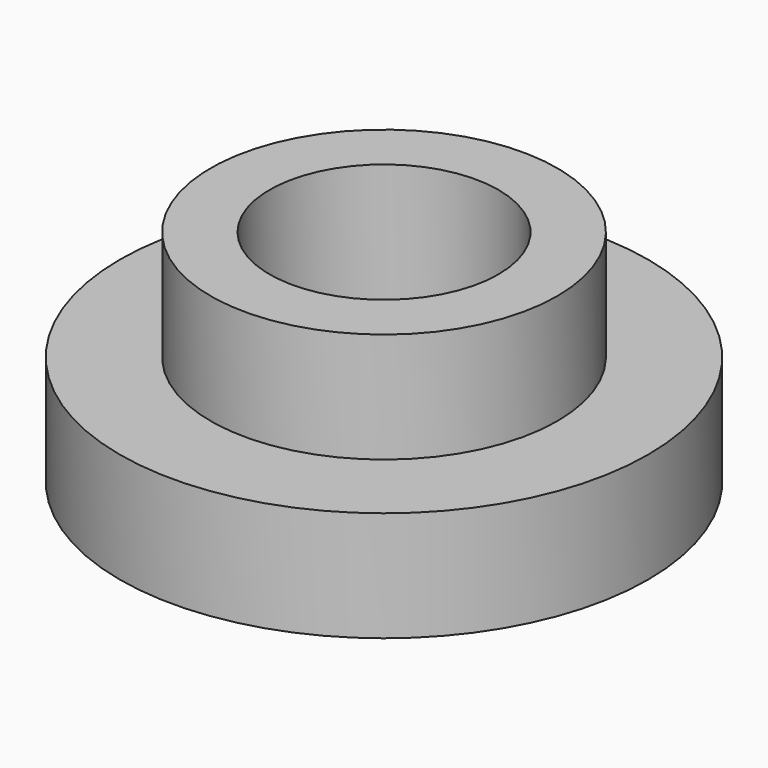
from build123d import *

# Parameters (mm, degrees)
F0_R     = 5
F1_DEPTH = 3.175
F2_R     = 7.62
F2_R_2   = 5
F3_DEPTH = 3.175
F4_R     = 3.302
F5_DEPTH = 6.351
F6_SIZE  = 0.381


with BuildPart() as f1:
    # F0 (on Top) → F1 (new body)
    with BuildSketch(Plane.XY):
        Circle(F0_R)
    extrude(amount=F1_DEPTH)

    # F2 (on face) → F3 (join)
    with BuildSketch(Plane(origin=(0, 0, 0), x_dir=(1, 0, 0), z_dir=(0, 0, -1))):
        Circle(F2_R)
        Circle(F2_R_2, mode=Mode.SUBTRACT)
        Circle(F2_R_2)
    extrude(amount=F3_DEPTH)

    # F4 (on face) → F5 (cut, through all)
    with BuildSketch(Plane.XY.offset(3.175)):
        Circle(F4_R)
    extrude(amount=-F5_DEPTH, mode=Mode.SUBTRACT)

    # F6
    f6_edges = [f1.edges().sort_by_distance(p)[0] for p in [
        (-3.302, 0, -3.175),
    ]]
    chamfer(f6_edges, length=F6_SIZE)


solid = f1.part
